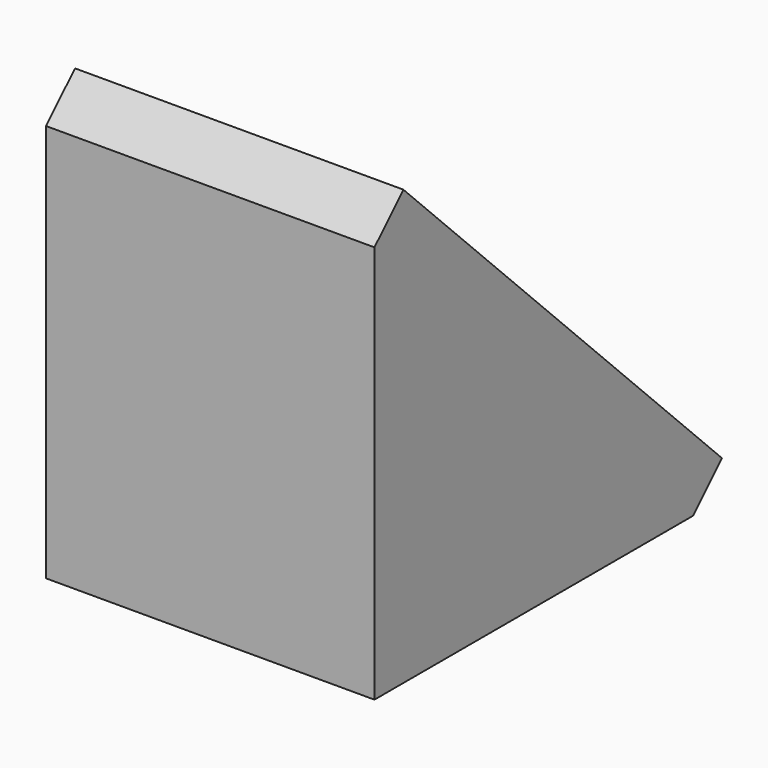
from build123d import *

# Parameters (mm, degrees)
F1_DEPTH = 18
F2_T     = -2.2
F4_DEPTH = 18
F3_W     = 13.6
F3_H     = 14.9906637612
F5_DEPTH = 8.9
F6_DEPTH = 2.8


# Not quite as in the source:
# - a feature of the source that left no trace in its solid (it failed there, or was rolled back) is left out


with BuildPart() as f1:
    # F0 (on Right) → F1 (new body)
    with BuildSketch(Plane.YZ):
        Polygon((0, 15), (0, 0), (15, 0), align=None)
    extrude(amount=F1_DEPTH)

    # F2
    f2_openings = [f1.faces().sort_by_distance(p)[0] for p in [
        (9, 7.5, 7.5),
    ]]
    offset(amount=F2_T, openings=f2_openings)

    # F0 (on Right) → F4 (join)
    with BuildSketch(Plane.YZ):
        Polygon((15, 0), (0, 0), (0, 15), (2.8284271247, 15), (-2, 19.8284271247), (-2, -2), (19.8284271247, -2), (15, 2.8284271247), align=None)
        Polygon((0, 15), (15, 0), (15, 2.8284271247), (2.8284271247, 15), align=None)
    extrude(amount=F4_DEPTH)

    # F3 (on face) → F5 (cut)
    with BuildSketch(Plane(origin=(0, 7.5, 7.5), x_dir=(1, 0, 0), z_dir=(0, 0.7071067812, 0.7071067812))):
        with Locations((9, 0)):
            Rectangle(F3_W, F3_H)
    extrude(amount=F5_DEPTH, mode=Mode.SUBTRACT)

    # F6 (add): a face of the model
    f6_faces = [f1.faces().sort_by_distance(p)[0] for p in [
        (9, 19.5757454612, -1.7473183365),
    ]]
    extrude(f6_faces, amount=F6_DEPTH)


solid = f1.part
